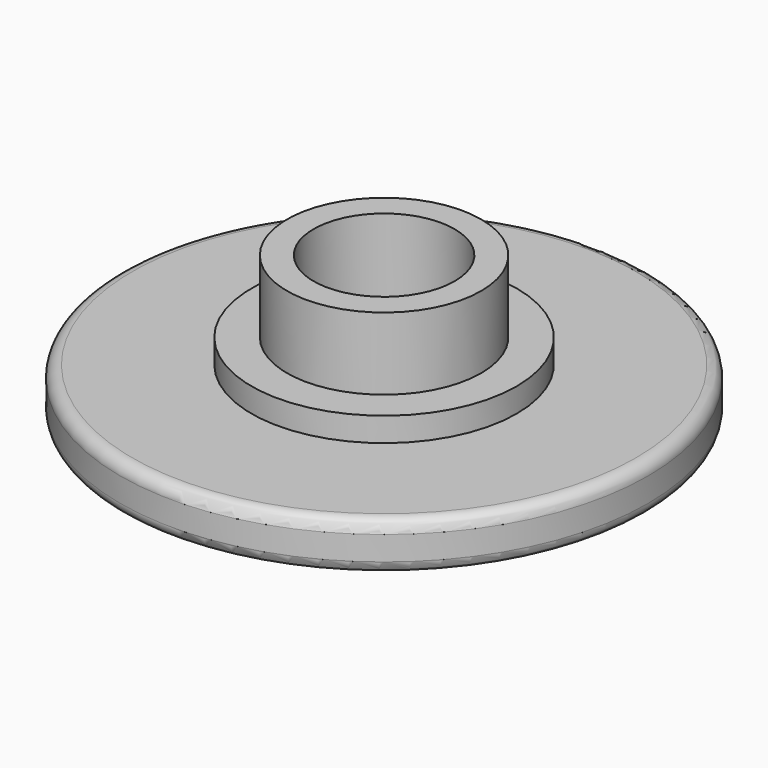
from build123d import *

# Parameters (mm, degrees)
F0_R         = 10.95
F0_R_2       = 0.069
F3_DEPTH     = 2
F1_R         = 5.5
F4_DEPTH     = 3
F2_R         = 4.025
F5_DEPTH     = 6
F6_R         = 0.5
F7_R         = 2.9249999207
F8_DEPTH     = 4
F9_TEXT_SIZE = 13.5641894303
F10_DEPTH    = 0.5


# Not quite as in the source:
# - Text() gives the source's letters only with a copy of the font that has no kerning and outlines rounded to 1/6400 em; it was checked with that copy


with BuildPart() as f3:
    # F0 (on Top) → F3 (new body)
    with BuildSketch(Plane.XY):
        Circle(F0_R)
        Circle(F0_R_2, mode=Mode.SUBTRACT)
    extrude(amount=F3_DEPTH)

    # F1 (on Top) → F4 (join)
    with BuildSketch(Plane.XY):
        Circle(F1_R)
    extrude(amount=F4_DEPTH)

    # F2 (on Top) → F5 (join)
    with BuildSketch(Plane.XY):
        Circle(F2_R)
    extrude(amount=F5_DEPTH)

    # F6
    f6_edges = [f3.edges().sort_by_distance(p)[0] for p in [
        (10.95, 0, 1),
        (-10.95, 0, 0),
        (-10.95, 0, 2),
    ]]
    fillet(f6_edges, radius=F6_R)

    # F7 (on face) → F8 (cut)
    with BuildSketch(Plane.XY.offset(6)):
        Circle(F7_R)
    extrude(amount=-F8_DEPTH, mode=Mode.SUBTRACT)

    # F9 (on face) → F10 (cut)
    with BuildSketch(Plane(origin=(0, 0, 0), x_dir=(1, 0, 0), z_dir=(0, 0, -1))):
        with Locations((-8.3012837567, -4.9940879107)):
            Text('DP', F9_TEXT_SIZE, font='Open Sans', font_style=FontStyle.ITALIC, text_align=(TextAlign.LEFT, TextAlign.BOTTOM))
    extrude(amount=-F10_DEPTH, mode=Mode.SUBTRACT)


solid = f3.part
